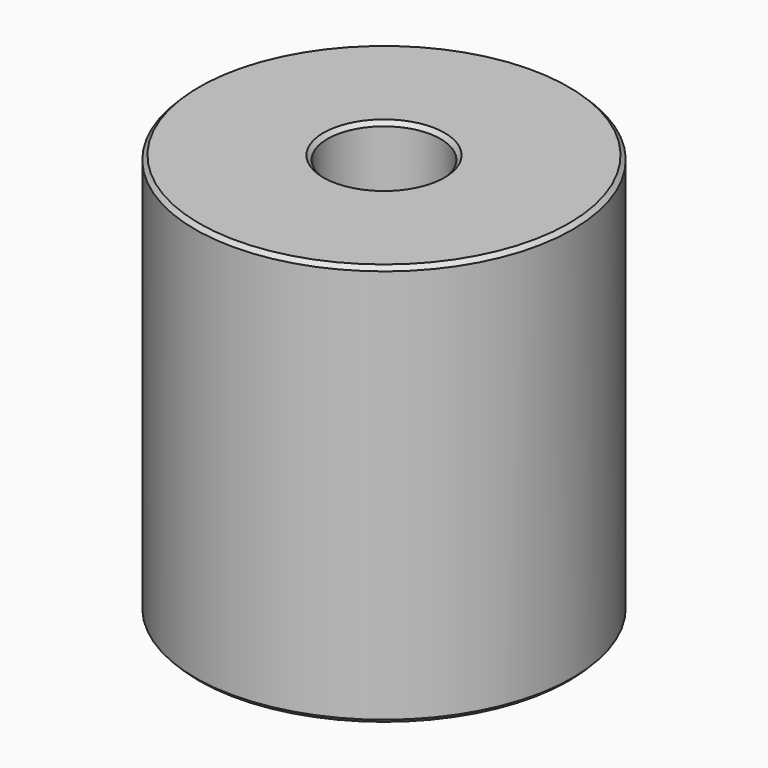
from build123d import *

# Parameters (mm, degrees)
F0_R           = 11.90625
F1_DEPTH       = 25.4
F2_D           = 7.1374
F2_CBORE_D     = 11.1125
F2_CBORE_DEPTH = 6.35
F3_SIZE        = 0.254


with BuildPart() as f1:
    # F0 (on Top) → F1 (new body)
    with BuildSketch(Plane.XY):
        Circle(F0_R)
    extrude(amount=F1_DEPTH)

    # F2 (through all)
    with Locations(Plane(origin=(0, 0, 0), x_dir=(1, 0, 0), z_dir=(0, 0, -1))):
        with Locations((0, 0)):
            CounterBoreHole(F2_D / 2, F2_CBORE_D / 2, F2_CBORE_DEPTH)

    # F3
    f3_edges = [f1.edges().sort_by_distance(p)[0] for p in [
        (-11.90625, 0, 25.4),
        (-11.90625, 0, 0),
        (-5.55625, 0, 0),
        (-3.5687, 0, 25.4),
    ]]
    chamfer(f3_edges, length=F3_SIZE)


solid = f1.part
